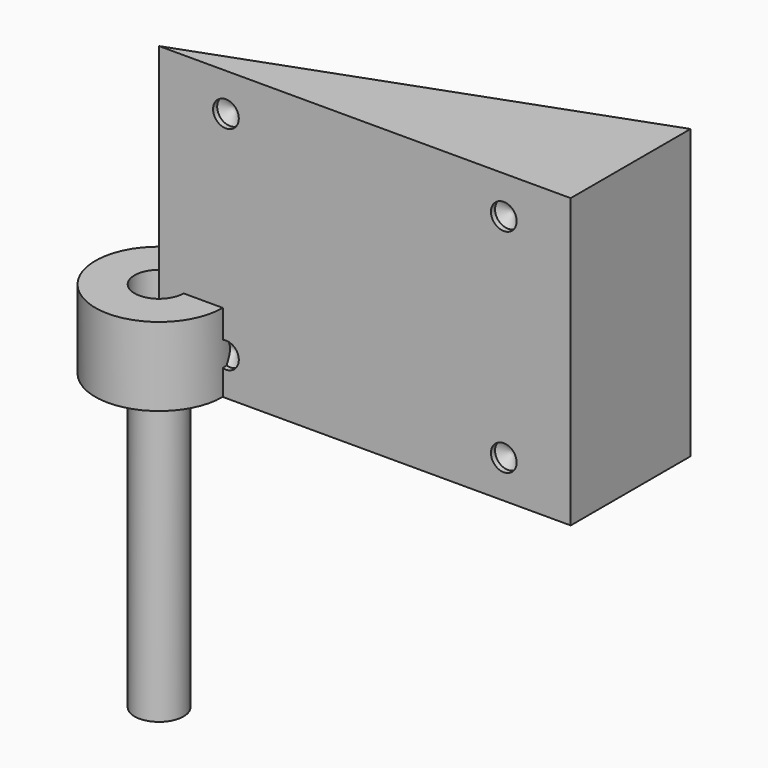
from build123d import *

# Parameters (mm, degrees)
F0_R           = 12.3825
F0_R_2         = 4.7625
F1_DEPTH       = 15.24
F2_R           = 4.7625
F3_DEPTH       = 5.953125
F4_DEPTH       = 57.15
F6_DEPTH       = 56
F9_D           = 5
F9_DEPTH       = 1
F9_TIP         = 1.5021515476
F9_ON_F8_D     = 5
F9_ON_F8_DEPTH = 1
F9_ON_F8_TIP   = 1.5021515476


# Not quite as in the source:
# - a length typed as a fraction of an inch, garbled in the dataset ("3 / 203.2 mm" for 3/8 in), is restored


with BuildPart() as f1:
    # F0 (on Top) → F1 (new body)
    with BuildSketch(Plane.XY):
        Circle(F0_R)
        Circle(F0_R_2, mode=Mode.SUBTRACT)
    extrude(amount=F1_DEPTH)


with BuildPart() as f3:
    # F2 (on Top) → F3 (new body)
    with BuildSketch(Plane.XY):
        Polygon((-1.5688368276, -8.1045527951), (6.234330193, -5.4109289447), (7.8031670207, 2.6936238504), (1.5688368276, 8.1045527951), (-6.234330193, 5.4109289447), (-7.8031670207, -2.6936238504), align=None)
        Circle(F2_R, mode=Mode.SUBTRACT)
        Circle(F2_R)
    extrude(amount=F3_DEPTH)

    # F2 (on Top) → F4 (join)
    with BuildSketch(Plane.XY):
        Circle(F2_R)
    extrude(amount=-F4_DEPTH)


with BuildPart() as f6:
    # F5 (on Top) → F6 (new body)
    with BuildSketch(Plane.XY):
        Polygon((80, 29.1176187413), (0, 0), (80, 0), align=None)
    extrude(amount=F6_DEPTH)

    # F9
    with Locations(Plane(origin=(0, 0, 0), x_dir=(-0.9396926208, -0.3420201433, 0), z_dir=(-0.3420201433, 0.9396926208, 0))):
        with Locations((-15.567110899, 48.6375), (-15.567110899, 7.3625), (-69.567110899, 7.3625), (-69.567110899, 48.6375)):
            Hole(F9_D / 2, depth=F9_DEPTH)
            with Locations((0, 0, -(F9_DEPTH + F9_TIP / 2))):  # 118° drill point
                Cone(0, F9_D / 2, F9_TIP, mode=Mode.SUBTRACT)

    # F9 on F8
    with Locations(Plane.XZ):
        with Locations((13, 48.6375), (13, 7.3625), (67, 48.6375), (67, 7.3625)):
            Hole(F9_ON_F8_D / 2, depth=F9_ON_F8_DEPTH)
            with Locations((0, 0, -(F9_ON_F8_DEPTH + F9_ON_F8_TIP / 2))):  # 118° drill point
                Cone(0, F9_ON_F8_D / 2, F9_ON_F8_TIP, mode=Mode.SUBTRACT)


solid = Compound([f1.part, f3.part, f6.part])
